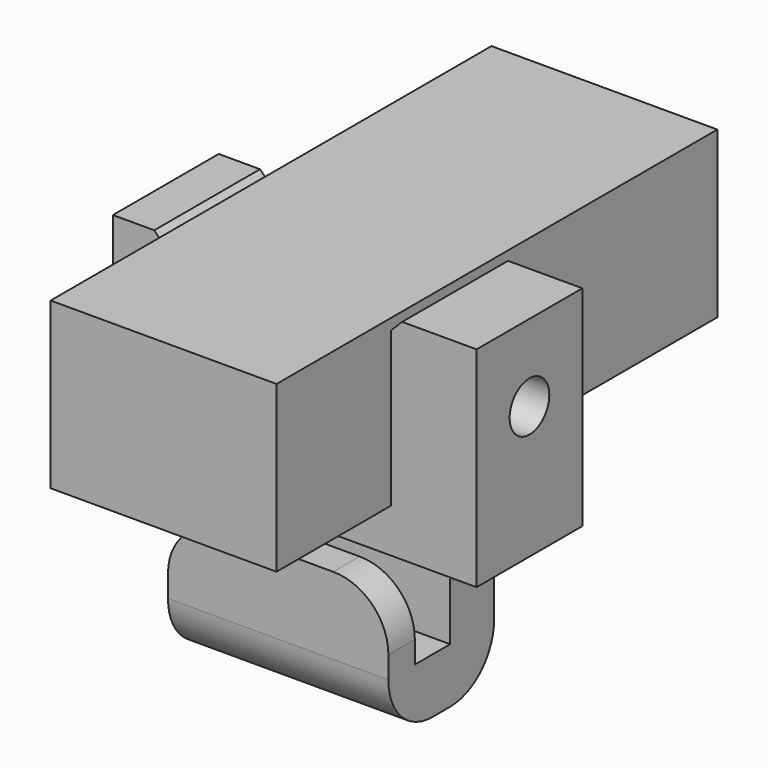
from build123d import *

# Parameters (mm, degrees)
F0_W          = 20.5
F0_H          = 15
F1_DEPTH      = 25
F1_DEPTH_BACK = 25
F3_DEPTH      = 12
F4_R          = 2.25
F5_DEPTH      = 7.75
F6_R          = 2.25
F7_DEPTH      = 3
F8_SIZE       = 1
F9_W          = 20
F9_H          = 15
F10_DEPTH     = 5
F11_W         = 20
F11_H         = 5
F12_DEPTH     = 7
F13_W         = 20
F13_H         = 3
F14_DEPTH     = 7
F15_R         = 4.99999


# Not quite as in the source:
# - a fillet or chamfer is up to 0.001 mm smaller than in the source, because OpenCascade refuses the exact size


with BuildPart() as f1:
    # F0 (on Front) → F1 (new body, two sides)
    with BuildSketch(Plane.XZ) as f1_sk:
        with Locations((0, 16.9023849815)):
            Rectangle(F0_W, F0_H)
    extrude(amount=F1_DEPTH)
    extrude(f1_sk.sketch, amount=-F1_DEPTH_BACK)


with BuildPart() as f3:
    # F2 (on Front) → F3 (new body)
    with BuildSketch(Plane.XZ):
        Polygon((-10.25, 24.4023849815), (-15, 24.4023849815), (-15, 5.4023849815), (18, 5.4023849815), (18, 24.4023849815), (10.25, 24.4023849815), (10.25, 9.4023849815), (-10.25, 9.4023849815), align=None)
    extrude(amount=F3_DEPTH)

    # F4 (on face) → F5 (cut, through all)
    with BuildSketch(Plane.YZ.offset(18)):
        with Locations((-6, 17.4023849815)):
            Circle(F4_R)
    extrude(amount=-F5_DEPTH, mode=Mode.SUBTRACT)

    # F6 (on face) → F7 (cut)
    with BuildSketch(Plane(origin=(10.25, 0, 0), x_dir=(0, -1, 0), z_dir=(-1, 0, 0))):
        Polygon((9.75, 19.567448491), (6, 21.7325120004), (2.25, 19.567448491), (2.25, 15.2373214721), (6, 13.0722579626), (9.75, 15.2373214721), align=None)
        with Locations((6, 17.4023849815)):
            Circle(F6_R, mode=Mode.SUBTRACT)
    extrude(amount=-F7_DEPTH, mode=Mode.SUBTRACT)

    # F8
    f8_edges = [f3.edges().sort_by_distance(p)[0] for p in [
        (10.25, -6, 24.402385),
        (-10.25, -6, 24.402385),
    ]]
    chamfer(f8_edges, length=F8_SIZE)

    # F9 (on face) → F10 (join)
    with BuildSketch(Plane(origin=(0, 0, 0), x_dir=(-1, 0, 0), z_dir=(0, 1, 0))):
        with Locations((0, -2.0976150185)):
            Rectangle(F9_W, F9_H)
    extrude(amount=-F10_DEPTH)

    # F11 (on face) → F12 (join)
    with BuildSketch(Plane.XZ.offset(5)):
        with Locations((0, -7.0976150185)):
            Rectangle(F11_W, F11_H)
    extrude(amount=F12_DEPTH)

    # F13 (on face) → F14 (join)
    with BuildSketch(Plane.XY.offset(-4.5976150185)):
        with Locations((0, -10.5)):
            Rectangle(F13_W, F13_H)
    extrude(amount=F14_DEPTH)

    # F15 (radius 5 in the source; OpenCascade refuses exactly that, so slightly less here)
    f15_edges = [f3.edges().sort_by_distance(p)[0] for p in [
        (0, 0, -9.597615),
        (0, -12, -9.597615),
        (10, -10.5, 2.402385),
        (-10, -10.5, 2.402385),
        (10, -2.5, 5.402385),
        (-10, -2.5, 5.402385),
    ]]
    fillet(f15_edges, radius=F15_R)


solid = Compound([f1.part, f3.part])
